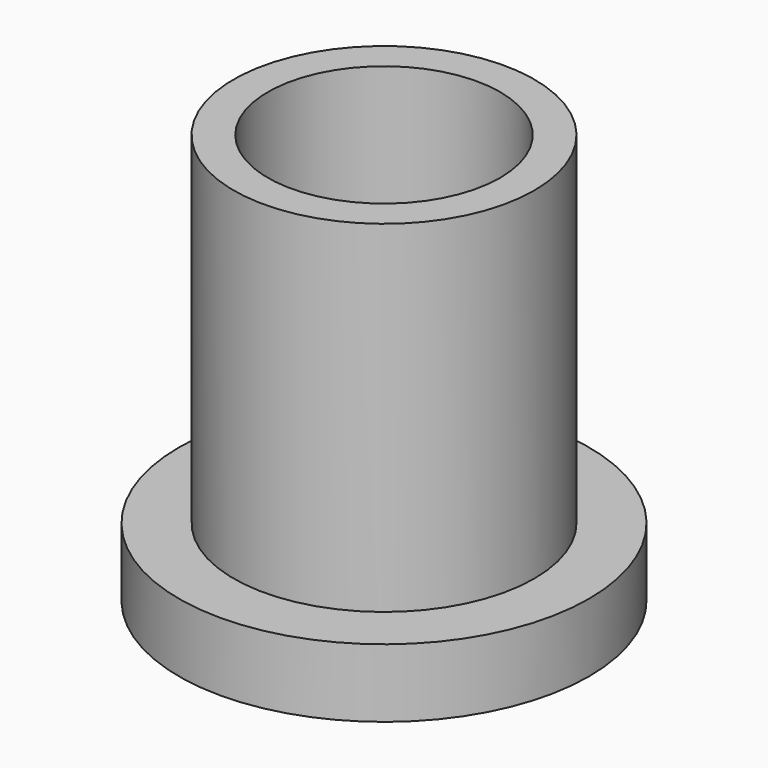
from build123d import *

# Parameters (mm, degrees)
F0_R     = 6
F0_R_2   = 4.4
F0_R_3   = 3.4
F1_DEPTH = 2
F2_DEPTH = 10
F3_DEPTH = 1.5
F4_DEPTH = 2


with BuildPart() as f1:
    # F0 (on Top) → F1 (new body)
    with BuildSketch(Plane.XY):
        Circle(F0_R)
        Circle(F0_R_2, mode=Mode.SUBTRACT)
        Circle(F0_R_2)
        Circle(F0_R_3, mode=Mode.SUBTRACT)
        Circle(F0_R_3)
        Polygon((0.8371578903, 1.45), (1.6743157806, 0), (0.8371578903, -1.45), (-0.8371578903, -1.45), (-1.6743157806, 0), (-0.8371578903, 1.45), align=None, mode=Mode.SUBTRACT)
    extrude(amount=-F1_DEPTH)

    # F0 (on Top) → F2 (join)
    with BuildSketch(Plane.XY):
        Circle(F0_R_2)
        Circle(F0_R_3, mode=Mode.SUBTRACT)
    extrude(amount=F2_DEPTH)

    # F0 (on Top) → F3 (join)
    with BuildSketch(Plane.XY):
        Polygon((0.8371578903, -1.45), (1.6743157806, 0), (0.8371578903, 1.45), (-0.8371578903, 1.45), (-1.6743157806, 0), (-0.8371578903, -1.45), align=None)
    extrude(amount=F3_DEPTH)

    # F4 (add): a face of the model
    f4_faces = [f1.faces().sort_by_distance(p)[0] for p in [
        (0, 0, 0),
    ]]
    extrude(f4_faces, amount=F4_DEPTH)


solid = f1.part
